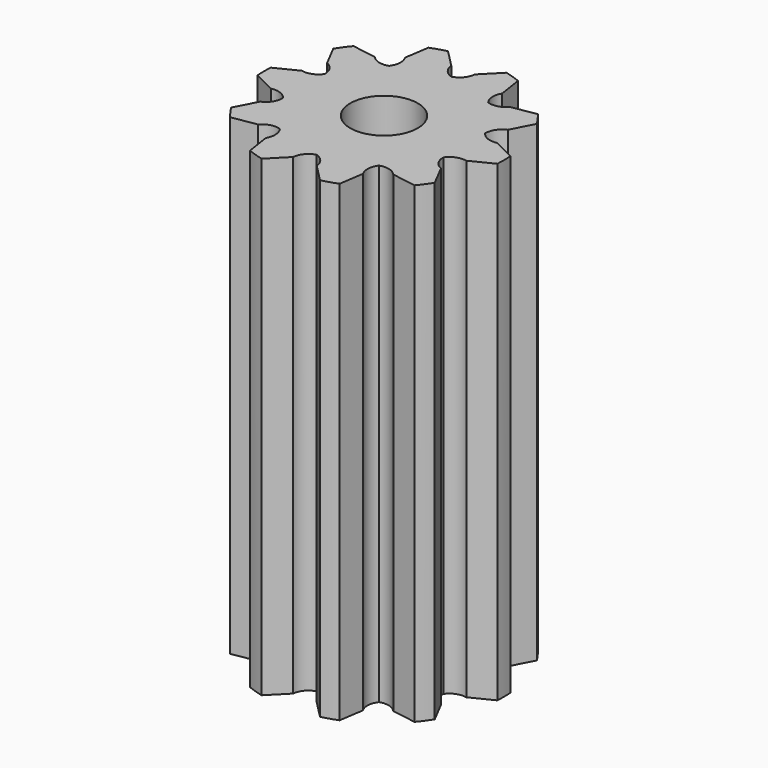
from build123d import *

# Parameters (mm, degrees)
F0_R     = 3.56
F1_DEPTH = 14
F2_R     = 1
F3_DEPTH = 20.5
F5_DEPTH = 14
F6_COUNT = 10


with BuildPart() as f1:
    # F0 (on Top) → F1 (new body)
    with BuildSketch(Plane.XY):
        Circle(F0_R)
    extrude(amount=F1_DEPTH)

    # F2 (on face) → F3 (cut)
    with BuildSketch(Plane.XY.offset(14)):
        Circle(F2_R)
    extrude(amount=-F3_DEPTH, mode=Mode.SUBTRACT)

    # F4 (on face) → F5 (cut)
    with BuildSketch(Plane.XY.offset(14)):
        with BuildLine():
            ThreePointArc((-0.3510643437, 2.9307105578), (-0.2410218301, 2.6619758494), (0, 2.5))
            ThreePointArc((0, 2.5), (0.2410218301, 2.6619758494), (0.3510643437, 2.9307105578))
            Line((0.3510643437, 2.9307105578), (0.8662797764, 3.4529928104))
            ThreePointArc((0.8662797764, 3.4529928104), (0, 3.56), (-0.8662797764, 3.4529928104))
            Line((-0.8662797764, 3.4529928104), (-0.3510643437, 2.9307105578))
        make_face()
    f5 = extrude(amount=-F5_DEPTH, mode=Mode.SUBTRACT)

    # F6: F5 ×10 about axis
    f6_axis = Axis((0, 0, 0), (0, 0, -1))
    for i in range(1, F6_COUNT):
        add(f5.rotate(f6_axis, i * 360 / F6_COUNT), mode=Mode.SUBTRACT)


solid = f1.part
